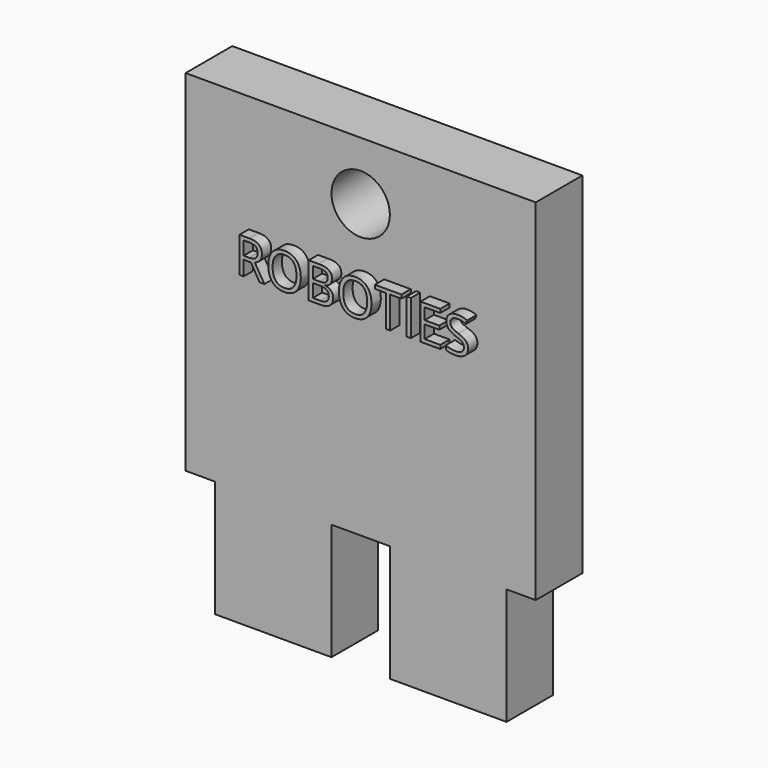
from build123d import *

# Parameters (mm, degrees)
F0_W         = 38.1
F0_H         = 50.8
F1_DEPTH     = 6.35
F2_R         = 3.175
F3_DEPTH     = 6.351
F4_W         = 3.175
F4_H         = 12.7
F5_DEPTH     = 6.351
F6_W         = 6.35
F6_H         = 12.7
F7_DEPTH     = 6.351
F8_TEXT_SIZE = 5.3897417194
F9_DEPTH     = 1.27


# Not quite as in the source:
# - Text() gives the source's letters only with a copy of the font that has no kerning and outlines rounded to 1/6400 em; it was checked with that copy


with BuildPart() as f1:
    # F0 (on Front) → F1 (new body)
    with BuildSketch(Plane.XZ):
        with Locations((-12.701960516, -33.3697550654)):
            Rectangle(F0_W, F0_H)
    extrude(amount=F1_DEPTH)

    # F2 (on face) → F3 (cut, through all)
    with BuildSketch(Plane.XZ.offset(6.35)):
        with Locations((-12.701960516, -14.3197550654)):
            Circle(F2_R)
    extrude(amount=-F3_DEPTH, mode=Mode.SUBTRACT)

    # F4 (on face) → F5 (cut, through all)
    with BuildSketch(Plane.XZ.offset(6.35)):
        with Locations((-30.164460516, -52.4197550654)):
            Rectangle(F4_W, F4_H)
        with Locations((4.760539484, -52.4197550654)):
            Rectangle(F4_W, F4_H)
    extrude(amount=-F5_DEPTH, mode=Mode.SUBTRACT)

    # F6 (on face) → F7 (cut, through all)
    with BuildSketch(Plane.XZ.offset(6.35)):
        with Locations((-12.701960516, -52.4197550654)):
            Rectangle(F6_W, F6_H)
    extrude(amount=-F7_DEPTH, mode=Mode.SUBTRACT)

    # F8 (on face) → F9 (join)
    with BuildSketch(Plane.XZ.offset(6.35)):
        with Locations((-25.4, -24.5503691034)):
            Text('ROBOTIES', F8_TEXT_SIZE, font='Open Sans', text_align=(TextAlign.LEFT, TextAlign.BOTTOM))
    extrude(amount=F9_DEPTH)


solid = f1.part
